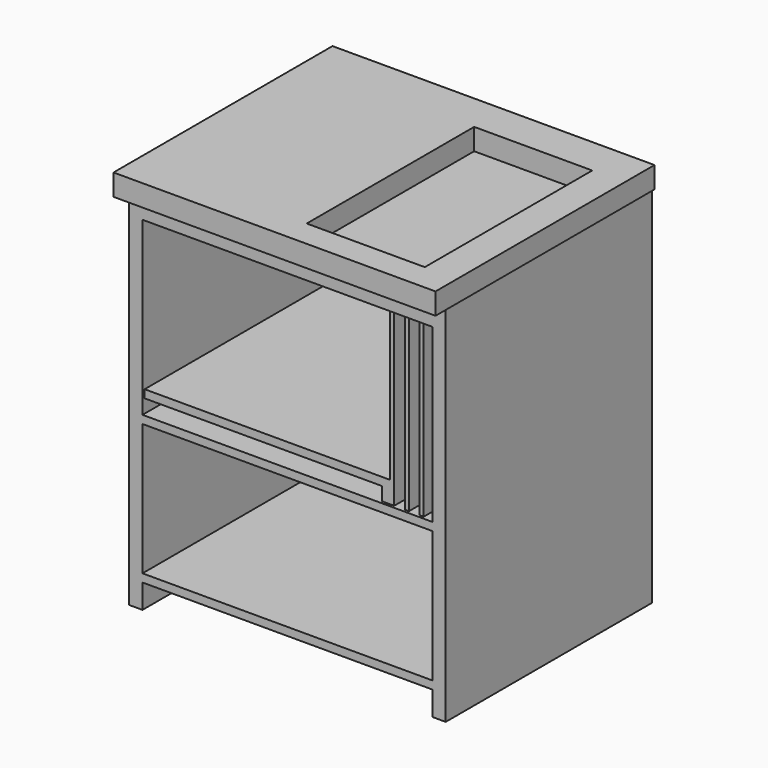
from build123d import *

# Parameters (mm, degrees)
F1_START = -38.1
F0_W     = 685.8
F0_H     = 19.05
F1_DEPTH = 609.6
F2_START = -44.45
F0_W_2   = 9.525
F0_H_2   = 406.4
F0_W_3   = 19.05
F0_H_3   = 31.75
F2_DEPTH = 603.25
F3_DEPTH = 647.7
F4_W     = 279.4
F4_H     = 495.3
F5_DEPTH = 914.401
F6_START = -38.1
F0_H_4   = 38.1
F6_DEPTH = 12.7


# Not quite as in the source:
# - a feature names something its author has since deleted; it is built from what else it names


with BuildPart() as f1:
    # F0 (on Front) → F1 (new body)
    with BuildSketch(Plane.XZ.offset(F1_START)):
        Polygon((-342.9, 355.6), (-374.65, 355.6), (-374.65, -457.2), (-342.9, -457.2), (-342.9, -400.05), (-342.9, -381), (-342.9, -69.85), (-342.9, -50.8), (-342.9, -19.05), (-342.9, 0), align=None)
        Polygon((342.9, -69.85), (342.9, -50.8), (317.5, -50.8), (307.975, -50.8), (282.575, -50.8), (273.05, -50.8), (247.65, -50.8), (238.125, -50.8), (219.075, -50.8), (-342.9, -50.8), (-342.9, -69.85), align=None)
        with Locations((0, -390.525)):
            Rectangle(F0_W, F0_H)
        Polygon((-342.9, 406.4), (-374.65, 406.4), (-374.65, 355.6), (-342.9, 355.6), (-342.9, 368.3), align=None)
        Polygon((374.65, 355.6), (374.65, 406.4), (342.9, 406.4), (342.9, 368.3), (342.9, 355.6), align=None)
        Polygon((-342.9, 368.3), (-342.9, 355.6), (238.125, 355.6), (247.65, 355.6), (273.05, 355.6), (282.575, 355.6), (307.975, 355.6), (317.5, 355.6), (342.9, 355.6), (342.9, 368.3), align=None)
        Polygon((374.65, -457.2), (374.65, 355.6), (342.9, 355.6), (342.9, -50.8), (342.9, -69.85), (342.9, -381), (342.9, -400.05), (342.9, -457.2), align=None)
    extrude(amount=-F1_DEPTH)

    # F0 (on Front) → F2 (join)
    with BuildSketch(Plane.XZ.offset(F2_START)):
        Polygon((247.65, 355.6), (238.125, 355.6), (238.125, 0), (238.125, -19.05), (238.125, -50.8), (247.65, -50.8), align=None)
        with Locations((277.8125, 152.4)):
            Rectangle(F0_W_2, F0_H_2)
        with Locations((312.7375, 152.4)):
            Rectangle(F0_W_2, F0_H_2)
        Polygon((238.125, 0), (-342.9, 0), (-342.9, -19.05), (219.075, -19.05), (238.125, -19.05), align=None)
        with Locations((228.6, -34.925)):
            Rectangle(F0_W_3, F0_H_3)
    extrude(amount=-F2_DEPTH)

    # F0 (on Front) → F6 (join)
    with BuildSketch(Plane.XZ.offset(F6_START)):
        with Locations((0, 387.35)):
            Rectangle(F0_W, F0_H_4)
    extrude(amount=-F6_DEPTH)


with BuildPart() as f3:
    # F0 (on Front) → F3 (new body, through all)
    with BuildSketch(Plane.XZ):
        Polygon((374.65, 457.2), (-374.65, 457.2), (-381, 457.2), (-381, 406.4), (-374.65, 406.4), (-342.9, 406.4), (342.9, 406.4), (374.65, 406.4), (381, 406.4), (381, 457.2), align=None)
    extrude(amount=-F3_DEPTH)

    # F4 (on face) → F5 (cut, through all)
    with BuildSketch(Plane.XY.offset(457.2)):
        with Locations((165.1, 311.15)):
            Rectangle(F4_W, F4_H)
    extrude(amount=-F5_DEPTH, mode=Mode.SUBTRACT)


solid = Compound([f1.part, f3.part])
